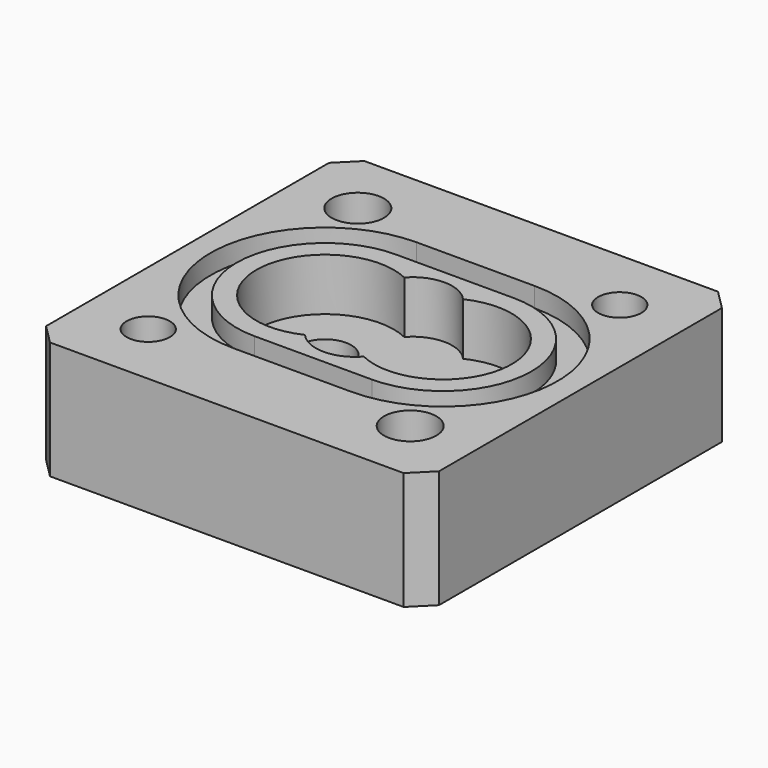
from build123d import *

# Parameters (mm, degrees)
F0_W     = 30
F0_H     = 30
F0_R     = 1.65
F0_R_2   = 2
F1_DEPTH = 9
F2_DEPTH = 1.5
F3_DEPTH = 7
F4_DEPTH = 4
F5_R     = 4
F5_R_2   = 2
F6_DEPTH = 1.5
F7_DEPTH = 10
F8_SIZE  = 1.5


# Not quite as in the source:
# - a feature names something its author has since deleted; it is built from what else it names


with BuildPart() as f1:
    # F0 (on Top) → F1 (new body)
    with BuildSketch(Plane.XY):
        with Locations((15, -15)):
            Rectangle(F0_W, F0_H)
        with Locations((5, -25)):
            Circle(F0_R, mode=Mode.SUBTRACT)
        with Locations((25, -25)):
            Circle(F0_R_2, mode=Mode.SUBTRACT)
        with Locations((5, -5)):
            Circle(F0_R_2, mode=Mode.SUBTRACT)
        with BuildLine():
            Line((19.5, -23.75), (10.5, -23.75))
            ThreePointArc((10.5, -23.75), (1.75, -15), (10.5, -6.25))
            Line((10.5, -6.25), (19.5, -6.25))
            ThreePointArc((19.5, -6.25), (28.25, -15), (19.5, -23.75))
        make_face(mode=Mode.SUBTRACT)
        with Locations((25, -5)):
            Circle(F0_R, mode=Mode.SUBTRACT)
        with BuildLine():
            ThreePointArc((10.5, -6.25), (1.75, -15), (10.5, -23.75))
            Line((10.5, -23.75), (19.5, -23.75))
            ThreePointArc((19.5, -23.75), (28.25, -15), (19.5, -6.25))
            Line((19.5, -6.25), (10.5, -6.25))
        make_face()
        with BuildLine():
            ThreePointArc((10.5, -21.75), (3.75, -15), (10.5, -8.25))
            Line((10.5, -8.25), (19.5, -8.25))
            ThreePointArc((19.5, -8.25), (26.25, -15), (19.5, -21.75))
            Line((19.5, -21.75), (10.5, -21.75))
        make_face(mode=Mode.SUBTRACT)
        with BuildLine():
            Line((19.5, -8.25), (10.5, -8.25))
            ThreePointArc((10.5, -8.25), (3.75, -15), (10.5, -21.75))
            Line((10.5, -21.75), (19.5, -21.75))
            ThreePointArc((19.5, -21.75), (26.25, -15), (19.5, -8.25))
        make_face()
        with BuildLine():
            ThreePointArc((17.2443308628, -10.25927677), (24.75, -15), (17.2443308628, -19.74072323))
            ThreePointArc((17.2443308628, -19.74072323), (15, -20.75), (12.7556691372, -19.74072323))
            ThreePointArc((12.7556691372, -19.74072323), (5.25, -15), (12.7556691372, -10.25927677))
            ThreePointArc((12.7556691372, -10.25927677), (15, -9.25), (17.2443308628, -10.25927677))
        make_face(mode=Mode.SUBTRACT)
        with BuildLine():
            ThreePointArc((12.7556691372, -19.74072323), (15, -20.75), (17.2443308628, -19.74072323))
            ThreePointArc((17.2443308628, -19.74072323), (24.75, -15), (17.2443308628, -10.25927677))
            ThreePointArc((17.2443308628, -10.25927677), (15, -9.25), (12.7556691372, -10.25927677))
            ThreePointArc((12.7556691372, -10.25927677), (5.25, -15), (12.7556691372, -19.74072323))
        make_face()
        with Locations((10.5, -15)):
            Circle(F0_R_2, mode=Mode.SUBTRACT)
        with Locations((19.5, -15)):
            Circle(F0_R_2, mode=Mode.SUBTRACT)
        with Locations((19.5, -15)):
            Circle(F0_R_2)
        with Locations((25, -25)):
            Circle(F0_R_2)
        with Locations((25, -5)):
            Circle(F0_R)
    extrude(amount=-F1_DEPTH)

    # F0 (on Top) → F2 (cut)
    with BuildSketch(Plane.XY):
        with BuildLine():
            ThreePointArc((10.5, -6.25), (1.75, -15), (10.5, -23.75))
            Line((10.5, -23.75), (19.5, -23.75))
            ThreePointArc((19.5, -23.75), (28.25, -15), (19.5, -6.25))
            Line((19.5, -6.25), (10.5, -6.25))
        make_face()
        with BuildLine():
            ThreePointArc((10.5, -21.75), (3.75, -15), (10.5, -8.25))
            Line((10.5, -8.25), (19.5, -8.25))
            ThreePointArc((19.5, -8.25), (26.25, -15), (19.5, -21.75))
            Line((19.5, -21.75), (10.5, -21.75))
        make_face(mode=Mode.SUBTRACT)
    extrude(amount=-F2_DEPTH, mode=Mode.SUBTRACT)

    # F0 (on Top) → F3 (cut)
    with BuildSketch(Plane.XY):
        with Locations((19.5, -15)):
            Circle(F0_R_2)
    extrude(amount=-F3_DEPTH, mode=Mode.SUBTRACT)

    # F0 (on Top) → F4 (cut)
    with BuildSketch(Plane.XY):
        with BuildLine():
            ThreePointArc((12.7556691372, -19.74072323), (15, -20.75), (17.2443308628, -19.74072323))
            ThreePointArc((17.2443308628, -19.74072323), (24.75, -15), (17.2443308628, -10.25927677))
            ThreePointArc((17.2443308628, -10.25927677), (15, -9.25), (12.7556691372, -10.25927677))
            ThreePointArc((12.7556691372, -10.25927677), (5.25, -15), (12.7556691372, -19.74072323))
        make_face()
        with Locations((10.5, -15)):
            Circle(F0_R_2, mode=Mode.SUBTRACT)
        with Locations((19.5, -15)):
            Circle(F0_R_2, mode=Mode.SUBTRACT)
    extrude(amount=-F4_DEPTH, mode=Mode.SUBTRACT)

    # F5 (on face) → F6 (cut)
    with BuildSketch(Plane(origin=(0, 0, -9), x_dir=(1, 0, 0), z_dir=(0, 0, -1))):
        with Locations((10.5, 15)):
            Circle(F5_R)
        with Locations((10.5, 15)):
            Circle(F5_R_2, mode=Mode.SUBTRACT)
    extrude(amount=-F6_DEPTH, mode=Mode.SUBTRACT)

    # F0 (on Top) → F7 (cut)
    with BuildSketch(Plane.XY):
        with Locations((25, -25)):
            Circle(F0_R_2)
        with Locations((25, -5)):
            Circle(F0_R)
    extrude(amount=-F7_DEPTH, mode=Mode.SUBTRACT)

    # F8
    f8_edges = [f1.edges().sort_by_distance(p)[0] for p in [
        (30, -30, -4.5),
        (30, 0, -4.5),
        (0, -30, -4.5),
        (0, 0, -4.5),
    ]]
    chamfer(f8_edges, length=F8_SIZE)


solid = f1.part
